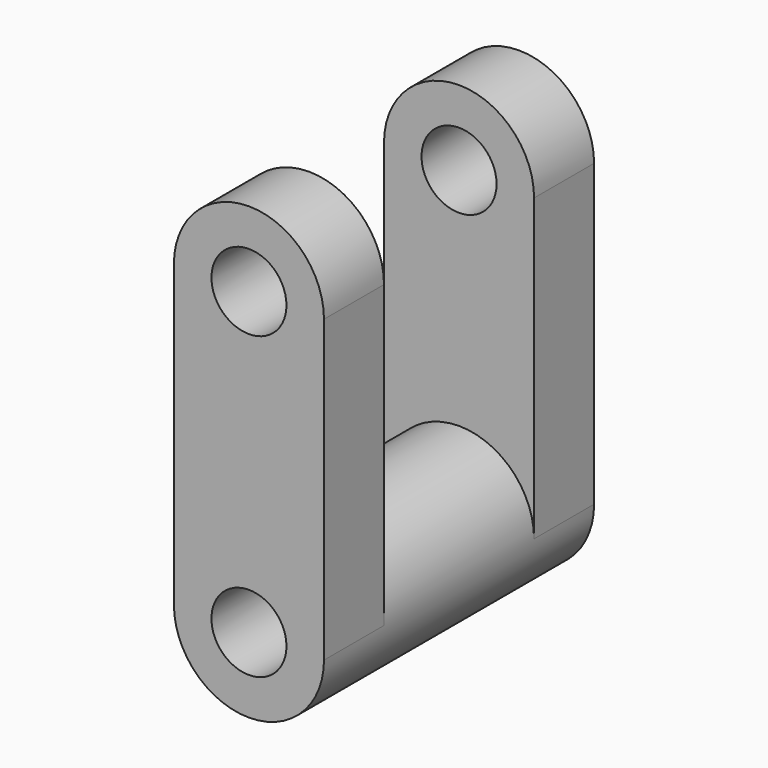
from build123d import *
from build123d import SkipClean  # not in build123d's __all__

# Parameters (mm, degrees)
F0_R     = 12.7
F1_DEPTH = 25.4
F2_R     = 25.4
F2_R_2   = 12.4458783194
F3_DEPTH = 63.5
F4_R     = 12.7
F5_DEPTH = 25.4


# Not quite as in the source:
# - after a boolean that leaves OpenCascade's solid faulty, fix() repairs it


with BuildPart() as f1:
    # F0 (on Front) → F1 (new body)
    with BuildSketch(Plane.XZ):
        with BuildLine():
            ThreePointArc((-25.4, -50.8), (0, -76.2), (25.4, -50.8))
            Line((25.4, -50.8), (25.4, 50.8))
            ThreePointArc((25.4, 50.8), (0, 76.2), (-25.4, 50.8))
            Line((-25.4, 50.8), (-25.4, -50.8))
        make_face()
        with Locations((0, -50.8)):
            Circle(F0_R, mode=Mode.SUBTRACT)
        with Locations((0, 50.8)):
            Circle(F0_R, mode=Mode.SUBTRACT)
    extrude(amount=-F1_DEPTH)

    # F2 (on face) → F3 (join)
    with BuildSketch(Plane.XZ):
        with Locations((0, -50.8)):
            Circle(F2_R)
        with Locations((0, -50.8)):
            Circle(F2_R_2, mode=Mode.SUBTRACT)
    with SkipClean():  # cleaning this boolean's faces spoils the solid; the shape is the same uncleaned
        extrude(amount=F3_DEPTH)

    # F4 (on face) → F5 (join)
    with BuildSketch(Plane.XZ.offset(63.5)):
        with BuildLine():
            Line((-25.4, 50.8), (-25.4, -50.8))
            ThreePointArc((-25.4, -50.8), (0, -25.4), (25.4, -50.8))
            Line((25.4, -50.8), (25.4, 50.8))
            ThreePointArc((25.4, 50.8), (0, 76.2), (-25.4, 50.8))
        make_face()
        with Locations((0, 50.8)):
            Circle(F4_R, mode=Mode.SUBTRACT)
        with BuildLine():
            ThreePointArc((25.4, -50.8), (0, -25.4), (-25.4, -50.8))
            ThreePointArc((-25.4, -50.8), (0, -76.2), (25.4, -50.8))
        make_face()
        with Locations((0, -50.8)):
            Circle(F4_R, mode=Mode.SUBTRACT)
    extrude(amount=F5_DEPTH)

    add(f1.part.fix(), mode=Mode.REPLACE)


solid = f1.part
